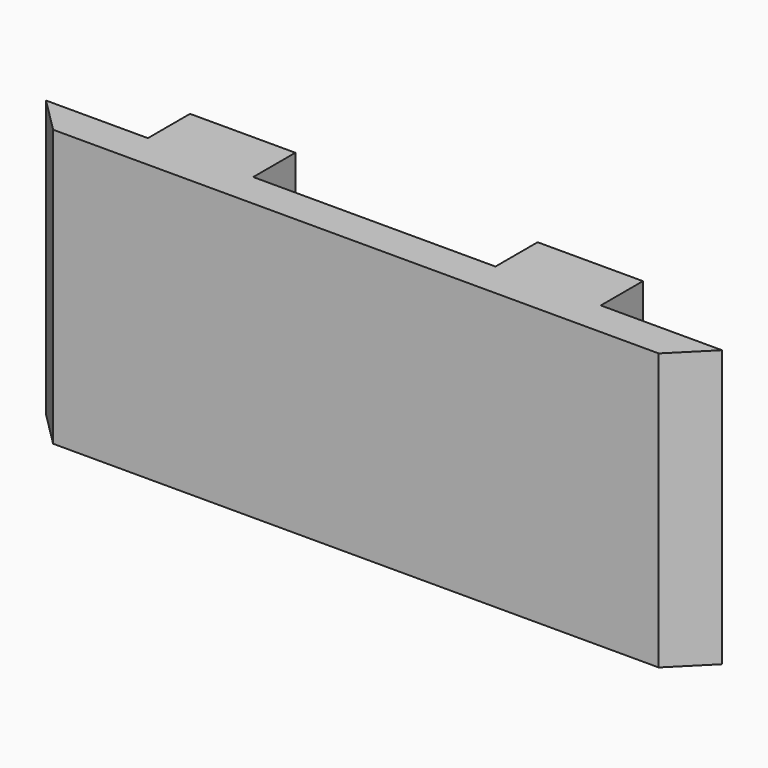
from build123d import *

# Parameters (mm, degrees)
F1_DEPTH  = 15.75
F3_D      = 4
F4_DEPTH  = 3
F5_W      = 3
F5_H      = 15.75
F6_DEPTH  = 25
F8_D      = 2
F9_W      = 6
F9_H      = 4
F10_DEPTH = 15.751
F11_SIZE  = 1
F12_SIZE  = 5
F13_DEPTH = 1
F14_DEPTH = 1
F15_W     = 0.1029567271
F15_H     = 11.4527670667
F15_W_2   = 37.000869453
F16_DEPTH = 15.751
F17_SIZE  = 1.99999


# Not quite as in the source:
# - a fillet or chamfer is up to 0.001 mm smaller than in the source, because OpenCascade refuses the exact size


with BuildPart() as f1:
    # F0 (on Top) → F1 (new body)
    with BuildSketch(Plane.XY):
        Polygon((0, 0), (44.5, 0), (44.5, 10), (37.6, 10), (37.6, 16), (31.6, 16), (31.6, 10), (17.8, 10), (17.8, 16), (11.8, 16), (11.8, 10), (0, 10), align=None)
    extrude(amount=F1_DEPTH)

    # F3 (through all)
    with Locations(Plane.XY.offset(15.75)):
        with Locations((24.7, 5)):
            Hole(F3_D / 2)

    # F4 (add): a face of the model
    f4_faces = [f1.faces().sort_by_distance(p)[0] for p in [
        (0, 5, 7.875),
    ]]
    extrude(f4_faces, amount=F4_DEPTH)

    # F5 (on face) → F6 (join)
    with BuildSketch(Plane(origin=(0, 10, 0), x_dir=(-1, 0, 0), z_dir=(0, 1, 0))):
        with Locations((1.5, 7.875)):
            Rectangle(F5_W, F5_H)
    extrude(amount=F6_DEPTH)

    # F8 (through all)
    with Locations(Plane.YZ):
        with Locations((27.25, 7.875), (17.75, 7.875)):
            Hole(F8_D / 2)

    # F9 (on face) → F10 (cut, through all)
    with BuildSketch(Plane.XY.offset(15.75)):
        with Locations((3, 8)):
            Rectangle(F9_W, F9_H)
    extrude(amount=-F10_DEPTH, mode=Mode.SUBTRACT)

    # F11
    f11_edges = [f1.edges().sort_by_distance(p)[0] for p in [
        (11.8, 16, 7.875),
        (17.8, 16, 7.875),
        (31.6, 16, 7.875),
        (37.6, 16, 7.875),
    ]]
    chamfer(f11_edges, length=F11_SIZE)

    # F12
    f12_edges = [f1.edges().sort_by_distance(p)[0] for p in [
        (44.5, 0, 7.875),
    ]]
    chamfer(f12_edges, length=F12_SIZE)

    # F13 (add): a face of the model
    f13_faces = [f1.faces().sort_by_distance(p)[0] for p in [
        (-3, 0.3838049635, 7.875),
    ]]
    extrude(f13_faces, amount=F13_DEPTH)

    # F14 (cut): a face of the model
    f14_faces = [f1.faces().sort_by_distance(p)[0] for p in [
        (0, 20.4721036707, 7.875),
    ]]
    extrude(f14_faces, amount=-F14_DEPTH, mode=Mode.SUBTRACT)

    # F15 (on face) → F16 (cut, through all)
    with BuildSketch(Plane.XY.offset(15.75)):
        with Locations((5.9485216364, 18.7263835333)):
            Rectangle(F15_W, F15_H)
        Polygon((6, 13), (5.8970432729, 13), (5.8970432729, 24.4527670667), (6, 24.4527670667), (6, 35.557191819), (-12.8509793431, 35.557191819), (-12.8509793431, -2.8801800217), (6, -2.8801800217), (6, 8), align=None)
        with Locations((24.5004347265, 18.7263835333)):
            Rectangle(F15_W_2, F15_H)
        Polygon((49.3548065424, 8), (6, 8), (6, -2.8801800217), (6, -4.4490518048), (49.3548065424, -4.4490518048), align=None)
    extrude(amount=-F16_DEPTH, mode=Mode.SUBTRACT)

    # F17 (size 2 in the source; OpenCascade refuses exactly that, so slightly less here)
    f17_edges = [f1.edges().sort_by_distance(p)[0] for p in [
        (6, 8, 7.875),
        (44.5, 8, 7.875),
    ]]
    chamfer(f17_edges, length=F17_SIZE)


solid = f1.part
